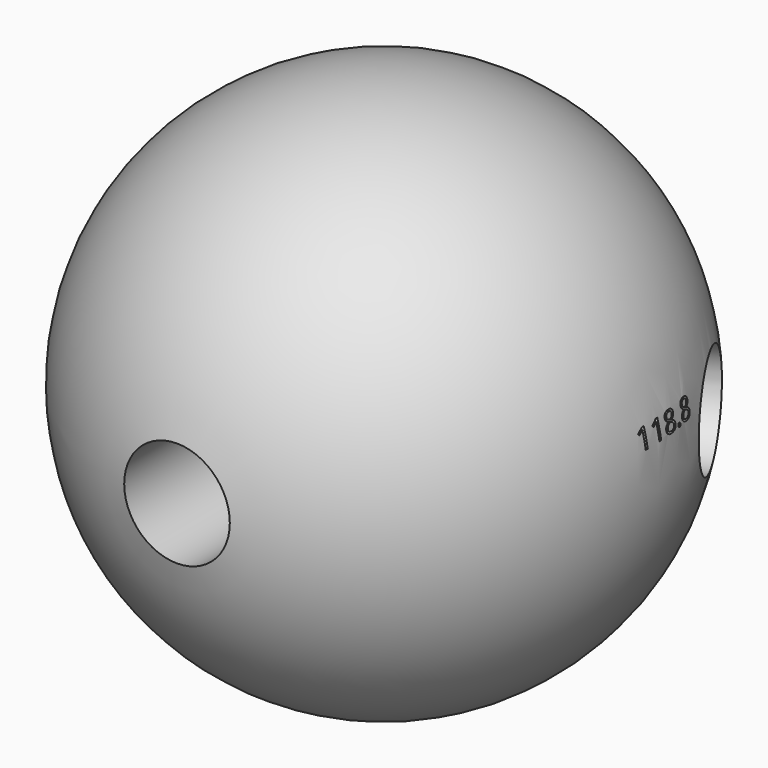
from build123d import *

# Parameters (mm, degrees)
F4_R            = 3.175
F5_DEPTH        = 25.4
F6_ANGLE        = -135.9
F7_ANGLE        = -105.3
F10_TEXT_SIZE   = 2.0451919732
F10_TEXT_SIZE_2 = 2.5728631752
F11_DEPTH       = 11.0236
F13_TEXT_SIZE   = 1.6643981022
F14_DEPTH       = 6.35


# Not quite as in the source:
# - Text() gives the source's letters only with a copy of the font that has no kerning and outlines rounded to 1/6400 em; it was checked with that copy


with BuildPart() as f1:
    # F0 (on Top) → F1 (revolve)
    with BuildSketch(Plane.XY):
        with BuildLine():
            Line((0, -15.875), (0, 15.875))
            ThreePointArc((0, 15.875), (-15.875, 0), (0, -15.875))
        make_face()
    revolve(axis=Axis((0, 0, 0), (0, -1, 0)))


with BuildPart() as f5:
    # F4 (on offset) → F5 (new body)
    with BuildSketch(Plane.XZ.offset(6.35)):
        Circle(F4_R)
    extrude(amount=F5_DEPTH)


with BuildPart() as f6_1:
    # F6: copy of F5
    add(f5.part.rotate(Axis((0, 0, 36.6811417043), (0, 0, 1)), F6_ANGLE))


with BuildPart() as f7_1:
    # F7: copy of F6_1
    add(f6_1.part.rotate(Axis((0, 0, 36.6811417043), (0, 0, 1)), F7_ANGLE))


with BuildPart() as f1_1:
    add(f1.part)

    # F8: cut F5, F6_1, F7_1
    add(f5.part, mode=Mode.SUBTRACT)
    add(f6_1.part, mode=Mode.SUBTRACT)
    add(f7_1.part, mode=Mode.SUBTRACT)

    # F10 (on offset) → F11 (cut)
    with BuildSketch(Plane(origin=(-13.0980531098, 13.5161423007, 0), x_dir=(-0.7181262978, -0.6959127966, 0), z_dir=(-0.6959127966, 0.7181262978, 0))):
        with Locations((-10.2289309725, 1.6021841438)):
            Text('105.3', F10_TEXT_SIZE, font='Open Sans', text_align=(TextAlign.LEFT, TextAlign.BOTTOM))
        with Locations((3.9429552853, 1.021825592)):
            Text('135.9', F10_TEXT_SIZE_2, font='Open Sans', text_align=(TextAlign.LEFT, TextAlign.BOTTOM))
    extrude(amount=-F11_DEPTH, mode=Mode.SUBTRACT)

    # F13 (on offset) → F14 (cut)
    with BuildSketch(Plane(origin=(16.5155767375, 9.0795151451, 0), x_dir=(-0.4817536741, 0.87630668, 0), z_dir=(0.87630668, 0.4817536741, 0))):
        with Locations((-8.1042200327, 1.6659615794)):
            Text('118.8', F13_TEXT_SIZE, font='Open Sans', text_align=(TextAlign.LEFT, TextAlign.BOTTOM))
    extrude(amount=-F14_DEPTH, mode=Mode.SUBTRACT)


solid = f1_1.part
